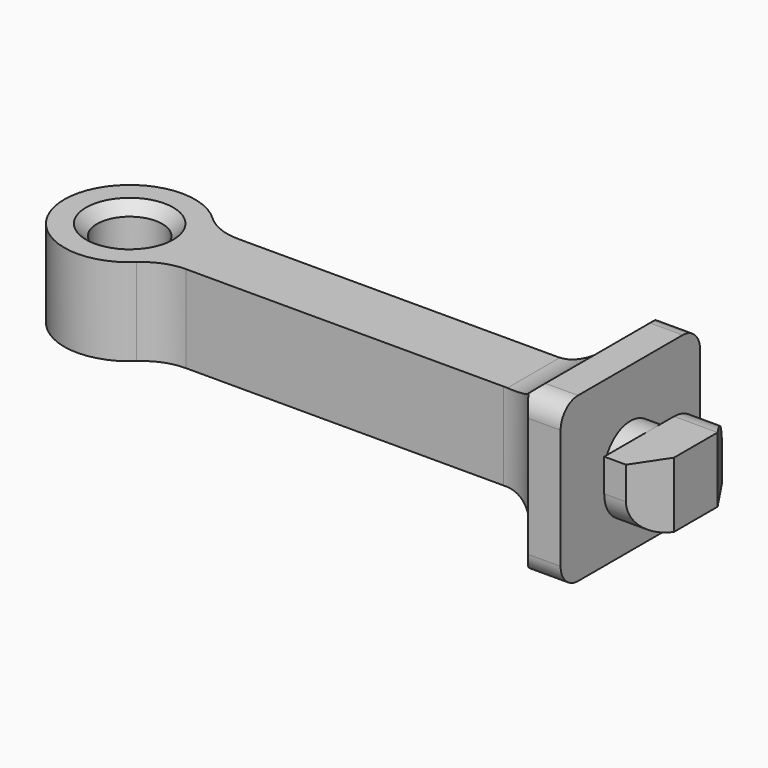
from build123d import *

# Parameters (mm, degrees)
F0_R      = 3
F1_DEPTH  = 15
F2_R      = 3
F3_DEPTH  = 2
F5_DEPTH  = 4
F7_DEPTH  = 25
F9_DEPTH  = 25
F11_DEPTH = 25
F12_SIZE  = 1
F13_SIZE  = 1
F14_R     = 2
F15_R     = 2
F16_R     = 3


# Not quite as in the source:
# - a feature names something its author has since deleted; it is built from what else it names


with BuildPart() as f1:
    # F0 (on Top) → F1 (new body)
    with BuildSketch(Plane.XY):
        with BuildLine():
            ThreePointArc((-38.3954955959, 25.79224433), (-40.2418679606, 26.1456424436), (-41.8272385211, 27.1558806937))
            ThreePointArc((-41.8272385211, 27.1558806937), (-51.9453300312, 22.79224433), (-41.8272385211, 18.4286079664))
            ThreePointArc((-41.8272385211, 18.4286079664), (-40.2418679606, 19.4388462165), (-38.3954955959, 19.79224433))
            Line((-38.3954955959, 19.79224433), (-9.2304363188, 19.79224433))
            ThreePointArc((-9.2304363188, 19.79224433), (-6.9849852462, 19.2596764203), (-5.2178762474, 17.7754241224))
            Line((-5.2178762474, 17.7754241224), (-3, 14.79224433))
            Line((-3, 14.79224433), (0, 14.79224433))
            Line((0, 14.79224433), (0, 19.79224433))
            Line((0, 19.79224433), (0, 25.79224433))
            Line((0, 25.79224433), (0, 30.79224433))
            Line((0, 30.79224433), (-3, 30.79224433))
            Line((-3, 30.79224433), (-5.2178762474, 27.8090645377))
            ThreePointArc((-5.2178762474, 27.8090645377), (-6.9849852462, 26.3248122398), (-9.2304363188, 25.79224433))
            Line((-9.2304363188, 25.79224433), (-38.3954955959, 25.79224433))
        make_face()
        with Locations((-45.9453300312, 22.79224433)):
            Circle(F0_R, mode=Mode.SUBTRACT)
    extrude(amount=F1_DEPTH)

    # F2 (on face) → F3 (join)
    with BuildSketch(Plane.YZ):
        with Locations((22.79224433, 7.5)):
            Circle(F2_R)
    extrude(amount=F3_DEPTH)

    # F4 (on face) → F5 (join)
    with BuildSketch(Plane.YZ.offset(2)):
        Polygon((17.29224433, 4.5), (26.29224433, 4.5), (28.29224433, 4.5), (28.29224433, 6), (28.29224433, 10.5), (19.29224433, 10.5), (17.29224433, 10.5), (17.29224433, 9), align=None)
    extrude(amount=F5_DEPTH)

    # F6 (on face) → F7 (cut)
    with BuildSketch(Plane(origin=(0, 0, 4.5), x_dir=(1, 0, 0), z_dir=(0, 0, -1))):
        Polygon((6, -17.29224433), (4, -17.29224433), (6, -20.29224433), align=None)
    extrude(amount=-F7_DEPTH, mode=Mode.SUBTRACT)

    # F8 (on face) → F9 (cut)
    with BuildSketch(Plane.XY.offset(10.5)):
        Polygon((6, 28.29224433), (4, 28.29224433), (6, 25.29224433), align=None)
    extrude(amount=-F9_DEPTH, mode=Mode.SUBTRACT)

    # F10 (on face) → F11 (cut)
    with BuildSketch(Plane.XZ.offset(-14.79224433)):
        with BuildLine():
            Line((-52.1873838902, 19.9649333954), (-52.1873838902, 11.5))
            Line((-52.1873838902, 11.5), (-8.8786755805, 11.5))
            ThreePointArc((-8.8786755805, 11.5), (-7.1200422145, 11.8194862799), (-5.5861525412, 12.7371165265))
            Line((-5.5861525412, 12.7371165265), (-3, 15))
            Line((-3, 15), (-3, 19.9649333954))
            Line((-3, 19.9649333954), (-52.1873838902, 19.9649333954))
        make_face()
        with BuildLine():
            Line((-2.2940631025, -5.0414614379), (-3, 0))
            Line((-3, 0), (-5.5861525412, 2.2628834735))
            ThreePointArc((-5.5861525412, 2.2628834735), (-7.1200422145, 3.1805137201), (-8.8786755805, 3.5))
            Line((-8.8786755805, 3.5), (-52.6222039647, 3.5))
            Line((-52.6222039647, 3.5), (-52.6222039647, -5.0414614379))
            Line((-52.6222039647, -5.0414614379), (-2.2940631025, -5.0414614379))
        make_face()
    extrude(amount=-F11_DEPTH, mode=Mode.SUBTRACT)

    # F12
    f12_edges = [f1.edges().sort_by_distance(p)[0] for p in [
        (-48.94533, 22.792244, 11.5),
    ]]
    chamfer(f12_edges, length=F12_SIZE)

    # F13
    f13_edges = [f1.edges().sort_by_distance(p)[0] for p in [
        (-48.94533, 22.792244, 3.5),
    ]]
    chamfer(f13_edges, length=F13_SIZE)

    # F14
    f14_edges = [f1.edges().sort_by_distance(p)[0] for p in [
        (-1.5, 14.792244, 15),
    ]]
    fillet(f14_edges, radius=F14_R)

    # F15
    f15_edges = [f1.edges().sort_by_distance(p)[0] for p in [
        (-1.5, 30.792244, 15),
        (-1.5, 30.792244, 0),
        (-1.5, 14.792244, 0),
    ]]
    fillet(f15_edges, radius=F15_R)

    # F16
    f16_edges = [f1.edges().sort_by_distance(p)[0] for p in [
        (3, 17.292244, 4.5),
        (3, 28.292244, 10.5),
    ]]
    fillet(f16_edges, radius=F16_R)


solid = f1.part
